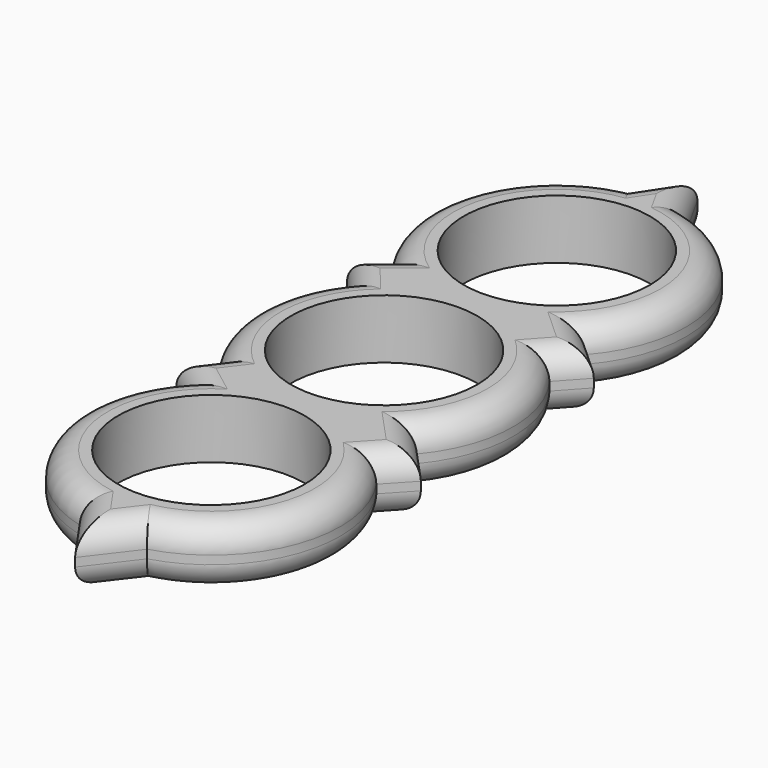
from build123d import *

# Parameters (mm, degrees)
F0_R     = 10.99185
F1_DEPTH = 7
F2_R     = 2.9999
F3_R     = 3


# Not quite as in the source:
# - a fillet or chamfer is up to 0.001 mm smaller than in the source, because OpenCascade refuses the exact size


with BuildPart() as f1:
    # F0 (on Top) → F1 (new body)
    with BuildSketch(Plane.XY):
        with BuildLine():
            Line((14.9749405682, 12.2164655477), (11.4485413794, 15.4244505109))
            ThreePointArc((11.4485413794, 15.4244505109), (14.496249252, 30.1865031666), (3.3629560629, 40.348023951))
            Line((3.3629560629, 40.348023951), (0.2675086434, 45.8798408508))
            Line((0.2675086434, 45.8798408508), (-3.3762647854, 40.3450066754))
            ThreePointArc((-3.3762647854, 40.3450066754), (-14.4677373847, 30.2734990528), (-11.5774462031, 15.5730824907))
            Line((-11.5774462031, 15.5730824907), (-14.7462384775, 12.9555240273))
            Line((-14.7462384775, 12.9555240273), (-11.90447345, 9.5153093422))
            ThreePointArc((-11.90447345, 9.5153093422), (-15.2385480834, -0.2103623294), (-11.6372767443, -9.8402942017))
            Line((-11.6372767443, -9.8402942017), (-14.0711786225, -13.0476644263))
            Line((-14.0711786225, -13.0476644263), (-11.2422357464, -15.194398011))
            ThreePointArc((-11.2422357464, -15.194398011), (-14.5942114147, -29.873072755), (-3.7012429532, -40.2674207969))
            Line((-3.7012429532, -40.2674207969), (0, -45.5736294389))
            Line((0, -45.5736294389), (4.1433280559, -40.1496617012))
            ThreePointArc((4.1433280559, -40.1496617012), (14.3389397361, -30.6462969476), (12.541204003, -16.8248431381))
            Line((12.541204003, -16.8248431381), (15.3642566875, -13.7878609821))
            Line((15.3642566875, -13.7878609821), (11.6764732619, -9.7937516899))
            ThreePointArc((11.6764732619, -9.7937516899), (15.2344796499, -0.4101582595), (12.1865310033, 9.1512874561))
            Line((12.1865310033, 9.1512874561), (14.9749405682, 12.2164655477))
        make_face()
        with Locations((0, -25.4837)):
            Circle(F0_R, mode=Mode.SUBTRACT)
        Circle(F0_R, mode=Mode.SUBTRACT)
        with Locations((0, 25.4837)):
            Circle(F0_R, mode=Mode.SUBTRACT)
    extrude(amount=F1_DEPTH)

    # F2 (radius 3 in the source; OpenCascade refuses exactly that, so slightly less here)
    f2_edges = [f1.edges().sort_by_distance(p)[0] for p in [
        (14.496249, 30.186503, 7),
        (-14.467737, 30.273499, 7),
        (1.815232, 43.113932, 7),
        (-1.554378, 43.112424, 7),
        (-13.325356, 11.235417, 7),
        (13.580736, 10.683877, 7),
        (15.23448, -0.410158, 7),
        (13.211741, 13.820458, 7),
        (-13.161842, 14.264303, 7),
        (-15.238548, -0.210362, 7),
        (-12.854228, -11.443979, 7),
        (-12.656707, -14.121031, 7),
        (13.520365, -11.790806, 7),
        (14.33894, -30.646297, 7),
        (13.95273, -15.306352, 7),
        (2.071664, -42.861646, 7),
        (-14.594211, -29.873073, 7),
        (-1.850621, -42.920525, 7),
    ]]
    fillet(f2_edges, radius=F2_R)

    # F3
    f3_edges = [f1.edges().sort_by_distance(p)[0] for p in [
        (-1.554378, 43.112424, 0),
        (-14.467737, 30.273499, 0),
        (1.815232, 43.113932, 0),
        (14.496249, 30.186503, 0),
        (-13.161842, 14.264303, 0),
        (13.211741, 13.820458, 0),
        (-13.325356, 11.235417, 0),
        (13.580736, 10.683877, 0),
        (-1.850621, -42.920525, 0),
        (-14.594211, -29.873073, 0),
        (2.071664, -42.861646, 0),
        (-12.656707, -14.121031, 0),
        (13.95273, -15.306352, 0),
        (-12.854228, -11.443979, 0),
        (13.520365, -11.790806, 0),
        (14.33894, -30.646297, 0),
        (-15.238548, -0.210362, 0),
        (15.23448, -0.410158, 0),
    ]]
    fillet(f3_edges, radius=F3_R)


solid = f1.part
